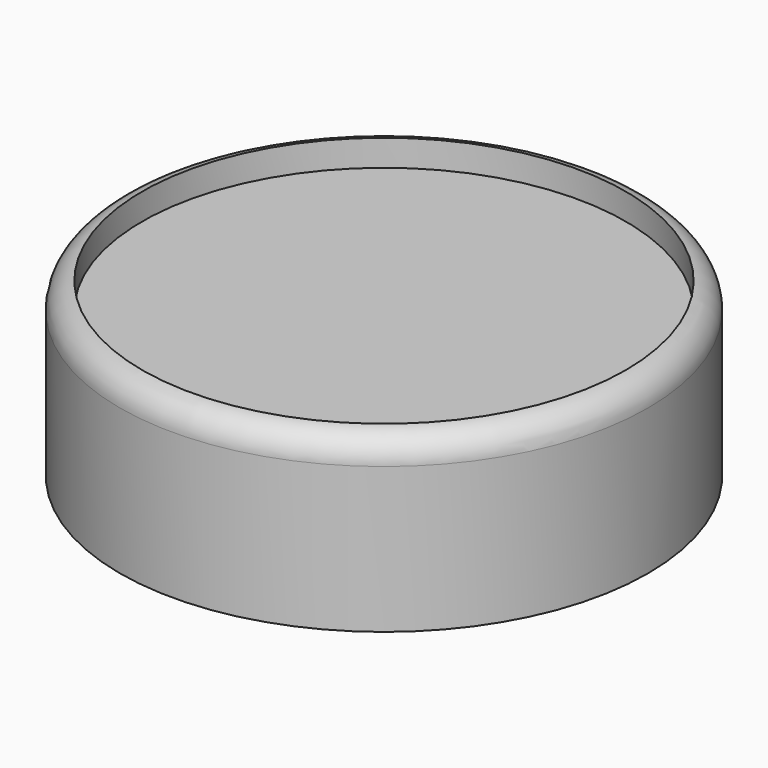
from build123d import *

# Parameters (mm, degrees)
F0_R     = 31.75
F1_DEPTH = 20.6375
F2_R     = 29.07284
F3_DEPTH = 3.175


# Not quite as in the source:
# - a fillet or chamfer that OpenCascade refuses, or shapes differently, is made with other operations: its cross-section is extruded or revolved along the edge and cut away or added


with BuildPart() as f1:
    # F0 (on Top) → F1 (new body)
    with BuildSketch(Plane.XY):
        Circle(F0_R)
    extrude(amount=F1_DEPTH)

    # F2 (on face) → F3 (cut)
    with BuildSketch(Plane.XY.offset(20.6375)):
        Circle(F2_R)
    extrude(amount=-F3_DEPTH, mode=Mode.SUBTRACT)

    # F4: fillet of radius 3.175 on 1 edges, made by hand

    # F4_s1 → F4_t2 (revolve, cut)
    with BuildSketch(Plane.XZ):
        with BuildLine():
            ThreePointArc((31.75, 17.5017735556), (30.9896704744, 19.5633243068), (29.07284, 20.6375))
            Line((29.07284, 20.6375), (31.75, 20.6375))
            Line((31.75, 20.6375), (31.75, 17.5017735556))
        make_face()
    revolve(axis=Axis((0, 0, 20.6375), (0, 0, 1)), mode=Mode.SUBTRACT)


solid = f1.part
